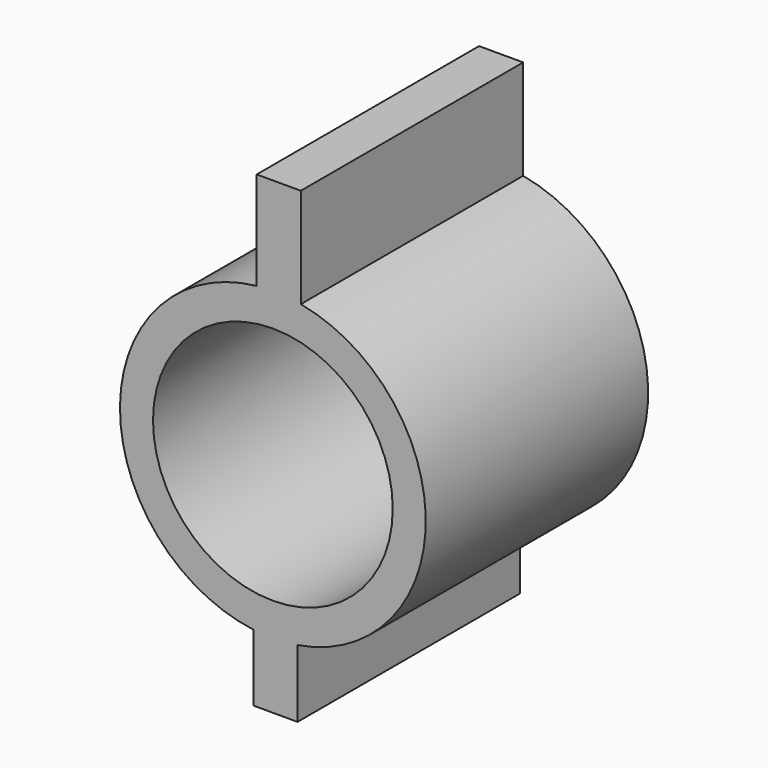
from build123d import *

# Parameters (mm, degrees)
F1_DEPTH = 63.5
F2_R     = 27.3812
F3_DEPTH = 101.6


# Not quite as in the source:
# - a feature names something its author has since deleted; it is built from what else it names


with BuildPart() as f1:
    # F0 (on Front) → F1 (new body)
    with BuildSketch(Plane.XZ):
        with BuildLine():
            ThreePointArc((-3.7017028225, 34.7282740892), (1.3544064685, 34.8987278868), (6.3820971775, 34.3369256139))
            Line((6.3820971775, 34.3369256139), (6.3820971775, 57.1461256139))
            Line((6.3820971775, 57.1461256139), (-3.7017028225, 57.1461256139))
            Line((-3.7017028225, 57.1461256139), (-3.7017028225, 34.7282740892))
        make_face()
        with BuildLine():
            Line((5.6386164435, -49.9173291028), (5.6386164435, -34.4668192557))
            ThreePointArc((5.6386164435, -34.4668192557), (0.6030353105, -34.9197934332), (-4.4451835565, -34.6409579566))
            Line((-4.4451835565, -34.6409579566), (-4.4451835565, -49.9173291028))
            Line((-4.4451835565, -49.9173291028), (5.6386164435, -49.9173291028))
        make_face()
        with BuildLine():
            ThreePointArc((5.6386164435, -34.4668192557), (26.6146980472, -22.6144527428), (34.925, 0))
            ThreePointArc((34.925, 0), (26.8574977327, 22.3255557722), (6.3820971775, 34.3369256139))
            ThreePointArc((6.3820971775, 34.3369256139), (1.3544064685, 34.8987278868), (-3.7017028225, 34.7282740892))
            ThreePointArc((-3.7017028225, 34.7282740892), (-34.9229942598, 0.3742952407), (-4.4451835565, -34.6409579566))
            ThreePointArc((-4.4451835565, -34.6409579566), (0.6030353105, -34.9197934332), (5.6386164435, -34.4668192557))
        make_face()
    extrude(amount=F1_DEPTH)

    # F2 (on face) → F3 (cut)
    with BuildSketch(Plane.XZ.offset(63.5)):
        Circle(F2_R)
    extrude(amount=-F3_DEPTH, mode=Mode.SUBTRACT)


solid = f1.part
